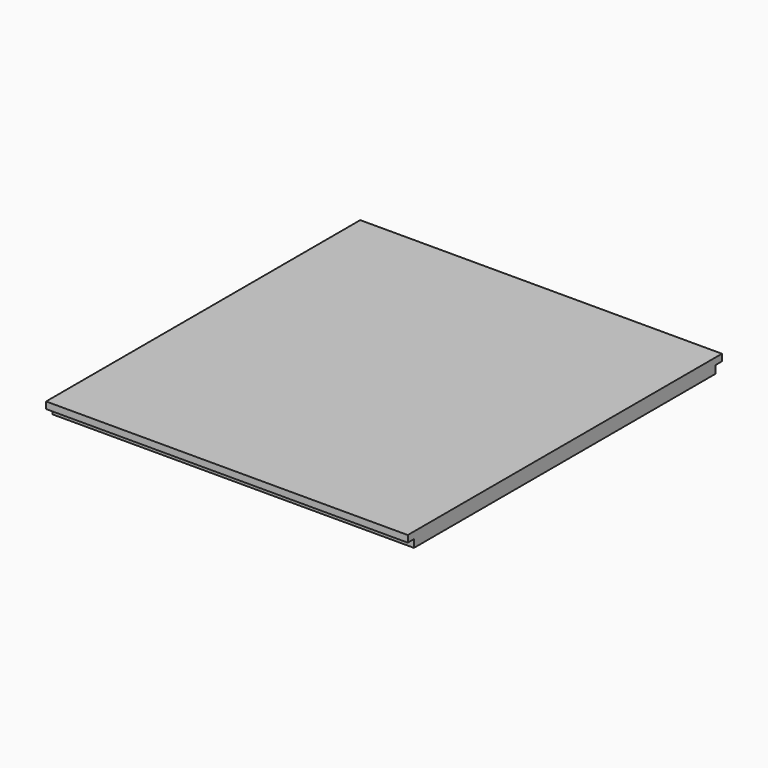
from build123d import *

# Parameters (mm, degrees)
F0_W     = 444.5
F0_H     = 482.6
F1_DEPTH = 17.78
F2_W     = 9.525
F2_H     = 9.525
F3_DEPTH = 444.5


# Not quite as in the source:
# - a feature of the source that left no trace in its solid (it failed there, or was rolled back) is left out


with BuildPart() as f1:
    # F0 (on Top) → F1 (new body)
    with BuildSketch(Plane.XY):
        with Locations((-25.2657681704, 0.1800126585)):
            Rectangle(F0_W, F0_H)
    extrude(amount=F1_DEPTH)

    # F2 (on face) → F3 (cut)
    with BuildSketch(Plane.YZ.offset(196.9842318296)):
        with Locations((236.7175126585, 4.7625)):
            Rectangle(F2_W, F2_H)
        with Locations((-236.3574873415, 4.7625)):
            Rectangle(F2_W, F2_H)
    extrude(amount=-F3_DEPTH, mode=Mode.SUBTRACT)


solid = f1.part
